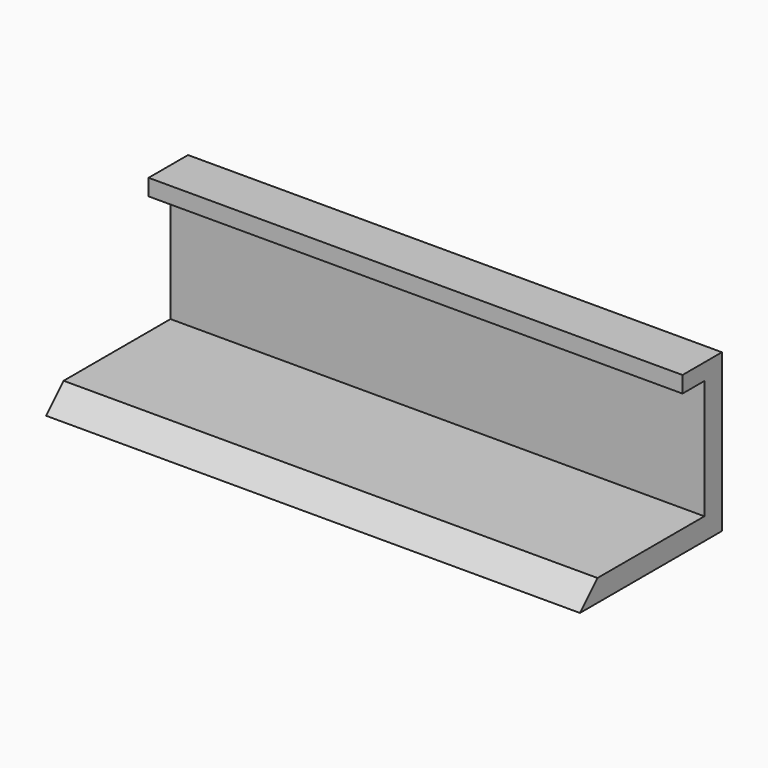
from build123d import *

# Parameters (mm, degrees)
F0_W     = 123.8177604973
F0_H     = 36.5064647049
F1_DEPTH = 5.08
F2_DEPTH = 4.826
F3_W     = 123.8177604973
F3_H     = 3.7974044681
F4_DEPTH = 6.35
F5_W     = 123.8177604973
F5_H     = 5.0793443806
F6_DEPTH = 36.068
F7_SIZE  = 5.079


# Not quite as in the source:
# - a fillet or chamfer is up to 0.001 mm smaller than in the source, because OpenCascade refuses the exact size


with BuildPart() as f1:
    # F0 (on Front) → F1 (new body)
    with BuildSketch(Plane.XZ):
        with Locations((4.7154184431, 8.8223954663)):
            Rectangle(F0_W, F0_H)
    extrude(amount=F1_DEPTH)

    # F0 (on Front) → F2 (join)
    with BuildSketch(Plane.XZ):
        with Locations((4.7154184431, 8.8223954663)):
            Rectangle(F0_W, F0_H)
    extrude(amount=F2_DEPTH)

    # F3 (on face) → F4 (join)
    with BuildSketch(Plane.XZ.offset(5.08)):
        with Locations((4.7154184431, 25.1769255847)):
            Rectangle(F3_W, F3_H)
    extrude(amount=F4_DEPTH)

    # F5 (on face) → F6 (join)
    with BuildSketch(Plane.XZ.offset(5.08)):
        with Locations((4.7154184431, -6.8911646958)):
            Rectangle(F5_W, F5_H)
    extrude(amount=F6_DEPTH)

    # F7 (size 5.08 in the source; OpenCascade refuses exactly that, so slightly less here)
    f7_edges = [f1.edges().sort_by_distance(p)[0] for p in [
        (4.715418, -41.148, -4.351493),
    ]]
    chamfer(f7_edges, length=F7_SIZE)


solid = f1.part
